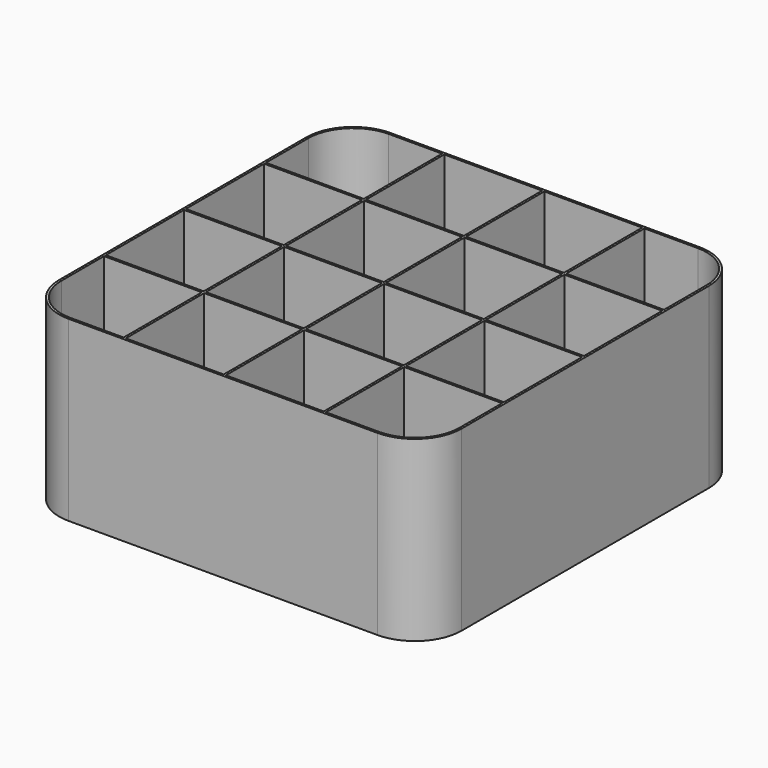
from build123d import *

# Parameters (mm, degrees)
F1_W         = 90.5
F1_H         = 90.5
F1_W_2       = 22
F1_H_2       = 22
F2_DEPTH     = 40
F4_DEPTH     = 0.6
F5_T1_DEPTH  = 40
F5_T6_DEPTH  = 64.4
F5_T11_DEPTH = 64.4
F6_R         = 10.5


# Not quite as in the source:
# - a fillet or chamfer that OpenCascade refuses, or shapes differently, is made with other operations: its cross-section is extruded or revolved along the edge and cut away or added


with BuildPart() as f2:
    # F1 (on Top) → F2 (new body)
    with BuildSketch(Plane.XY):
        with Locations((44.75, 44.75)):
            Rectangle(F1_W, F1_H)
        with Locations((11, 11)):
            Rectangle(F1_W_2, F1_H_2, mode=Mode.SUBTRACT)
        with Locations((33.5, 11)):
            Rectangle(F1_W_2, F1_H_2, mode=Mode.SUBTRACT)
        with Locations((11, 33.5)):
            Rectangle(F1_W_2, F1_H_2, mode=Mode.SUBTRACT)
        with Locations((33.5, 33.5)):
            Rectangle(F1_W_2, F1_H_2, mode=Mode.SUBTRACT)
        with Locations((56, 11)):
            Rectangle(F1_W_2, F1_H_2, mode=Mode.SUBTRACT)
        with Locations((78.5, 11)):
            Rectangle(F1_W_2, F1_H_2, mode=Mode.SUBTRACT)
        with Locations((56, 33.5)):
            Rectangle(F1_W_2, F1_H_2, mode=Mode.SUBTRACT)
        with Locations((78.5, 33.5)):
            Rectangle(F1_W_2, F1_H_2, mode=Mode.SUBTRACT)
        with Locations((11, 56)):
            Rectangle(F1_W_2, F1_H_2, mode=Mode.SUBTRACT)
        with Locations((33.5, 56)):
            Rectangle(F1_W_2, F1_H_2, mode=Mode.SUBTRACT)
        with Locations((11, 78.5)):
            Rectangle(F1_W_2, F1_H_2, mode=Mode.SUBTRACT)
        with Locations((33.5, 78.5)):
            Rectangle(F1_W_2, F1_H_2, mode=Mode.SUBTRACT)
        with Locations((56, 56)):
            Rectangle(F1_W_2, F1_H_2, mode=Mode.SUBTRACT)
        with Locations((78.5, 56)):
            Rectangle(F1_W_2, F1_H_2, mode=Mode.SUBTRACT)
        with Locations((56, 78.5)):
            Rectangle(F1_W_2, F1_H_2, mode=Mode.SUBTRACT)
        with Locations((78.5, 78.5)):
            Rectangle(F1_W_2, F1_H_2, mode=Mode.SUBTRACT)
    extrude(amount=F2_DEPTH)

    # F3 (on face) → F4 (join)
    with BuildSketch(Plane(origin=(0, 0, 0), x_dir=(1, 0, 0), z_dir=(0, 0, -1))):
        Polygon((22, -89.5), (22, -88.0857864376), (1.4142135624, -67.5), (0, -67.5), (0, -68.9142135624), (20.5857864376, -89.5), align=None)
        Polygon((22, -67), (22, -65.5857864376), (1.4142135624, -45), (0, -45), (0, -46.4142135624), (20.5857864376, -67), align=None)
        Polygon((44.5, -89.5), (44.5, -88.0857864376), (23.9142135624, -67.5), (22.5, -67.5), (22.5, -68.9142135624), (43.0857864376, -89.5), align=None)
        Polygon((22, -44.5), (22, -43.0857864376), (1.4142135624, -22.5), (0, -22.5), (0, -23.9142135624), (20.5857864376, -44.5), align=None)
        Polygon((44.5, -67), (44.5, -65.5857864376), (23.9142135624, -45), (22.5, -45), (22.5, -46.4142135624), (43.0857864376, -67), align=None)
        Polygon((67, -89.5), (67, -88.0857864376), (46.4142135624, -67.5), (45, -67.5), (45, -68.9142135624), (65.5857864376, -89.5), align=None)
        Polygon((89.5, -89.5), (89.5, -88.0857864376), (68.9142135624, -67.5), (67.5, -67.5), (67.5, -68.9142135624), (88.0857864376, -89.5), align=None)
        Polygon((67, -67), (67, -65.5857864376), (46.4142135624, -45), (45, -45), (45, -46.4142135624), (65.5857864376, -67), align=None)
        Polygon((44.5, -44.5), (44.5, -43.0857864376), (23.9142135624, -22.5), (22.5, -22.5), (22.5, -23.9142135624), (43.0857864376, -44.5), align=None)
        Polygon((22, -22), (22, -20.5857864376), (1.4142135624, 0), (0, 0), (0, -1.4142135624), (20.5857864376, -22), align=None)
        Polygon((22.5, -1.4142135624), (43.0857864376, -22), (44.5, -22), (44.5, -20.5857864376), (23.9142135624, 0), (22.5, 0), align=None)
        Polygon((45, -23.9142135624), (65.5857864376, -44.5), (67, -44.5), (67, -43.0857864376), (46.4142135624, -22.5), (45, -22.5), align=None)
        Polygon((67.5, -46.4142135624), (88.0857864376, -67), (89.5, -67), (89.5, -65.5857864376), (68.9142135624, -45), (67.5, -45), align=None)
        Polygon((67.5, -23.9142135624), (88.0857864376, -44.5), (89.5, -44.5), (89.5, -43.0857864376), (68.9142135624, -22.5), (67.5, -22.5), align=None)
        Polygon((45, -1.4142135624), (65.5857864376, -22), (67, -22), (67, -20.5857864376), (46.4142135624, 0), (45, 0), align=None)
        Polygon((67.5, -1.4142135624), (88.0857864376, -22), (89.5, -22), (89.5, -20.5857864376), (68.9142135624, 0), (67.5, 0), align=None)
    extrude(amount=-F4_DEPTH)

    # F5: fillet of radius 10 on 4 edges, made by hand

    # F5_s2 → F5_t1 (join)
    with BuildSketch(Plane.XY):
        with BuildLine():
            ThreePointArc((89.5, 10), (86.5710678119, 2.9289321881), (79.5, 0))
            Line((79.5, 0), (89.5, 0))
            Line((89.5, 0), (89.5, 10))
        make_face()
        with BuildLine():
            ThreePointArc((10, 89.5), (2.9289321881, 86.5710678119), (0, 79.5))
            Line((0, 79.5), (0, 89.5))
            Line((0, 89.5), (10, 89.5))
        make_face()
    extrude(amount=F5_T1_DEPTH)


with BuildPart() as f5_tool4:
    # F5_s5 → F5_t6 (new body)
    with BuildSketch(Plane.XY.offset(-24.4)):
        with BuildLine():
            ThreePointArc((0, 10), (2.9289321881, 2.9289321881), (10, 0))
            Line((10, 0), (0, 0))
            Line((0, 0), (0, 10))
        make_face()
    extrude(amount=F5_T6_DEPTH)

    split(bisect_by=Plane.XY, keep=Keep.TOP)


with BuildPart() as f2_1:
    add(f2.part)

    # F5_t3: union F5_tool4
    add(f5_tool4.part)


with BuildPart() as f5_tool9:
    # F5_s10 → F5_t11 (new body)
    with BuildSketch(Plane.XY.offset(-24.4)):
        with BuildLine():
            ThreePointArc((79.5, 89.5), (86.5710678119, 86.5710678119), (89.5, 79.5))
            Line((89.5, 79.5), (89.5, 89.5))
            Line((89.5, 89.5), (79.5, 89.5))
        make_face()
    extrude(amount=F5_T11_DEPTH)

    split(bisect_by=Plane.XY, keep=Keep.TOP)


with BuildPart() as f2_2:
    add(f2_1.part)

    # F5_t8: union F5_tool9
    add(f5_tool9.part)

    # F6
    f6_edges = [f2_2.edges().sort_by_distance(p)[0] for p in [
        (90, -0.5, 20),
        (-0.5, -0.5, 20),
        (-0.5, 90, 20),
        (90, 90, 20),
    ]]
    fillet(f6_edges, radius=F6_R)


solid = f2_2.part
